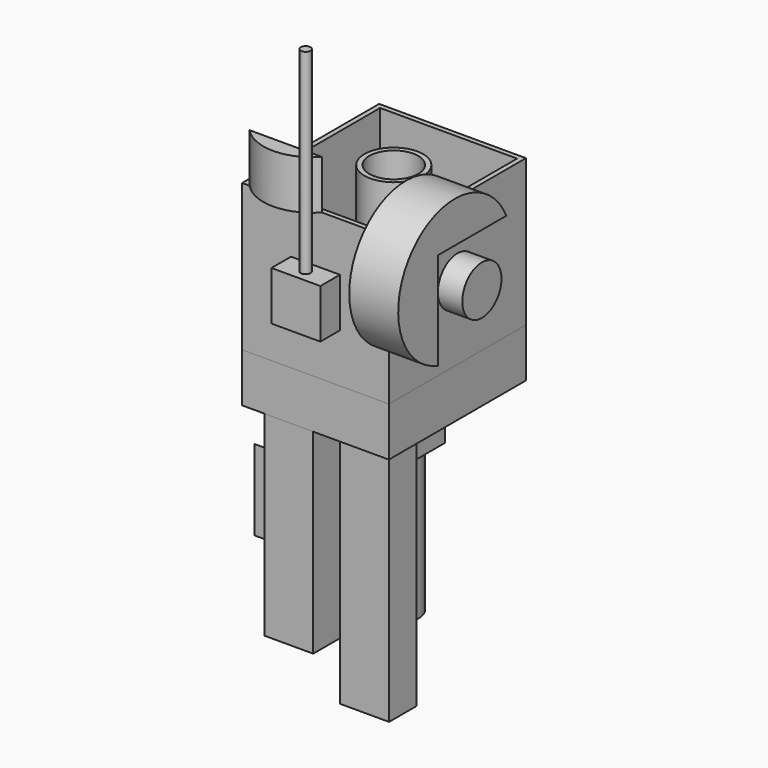
from build123d import *

# Parameters (mm, degrees)
F0_W          = 76.2
F0_H          = 76.2
F1_DEPTH      = 76.2
F3_D          = 25.4
F5_W          = 76.2
F5_H          = 76.2
F5_W_2        = 25.4
F5_H_2        = 25.4
F1_FACE1_W    = 76.2
F1_FACE1_H    = 76.2
F1_FACE2_W    = 76.2
F1_FACE2_H    = 76.2
F4_W          = 76.2
F4_H          = 76.2
F6_DEPTH      = 12.7
F7_W          = 25.4
F7_H          = 25.4
F8_DEPTH      = 12.7
F9_R          = 12.7
F10_DEPTH     = 12.7
F11_DEPTH     = 12.7
F14_DEPTH     = 25.4
F16_DEPTH     = 25.4
F17_R         = 2.54
F18_DEPTH     = 101.6
F21_W         = 25.4
F21_H         = 17.9451964796
F22_DEPTH     = 177.8
F23_W         = 25.4
F23_H         = 25.4
F24_DEPTH     = 127
F23_R         = 12.7
F25_DEPTH     = 25.4
F26_W         = 25.4
F26_H         = 25.4
F26_W_2       = 2.54
F26_H_2       = 2.54
F27_DEPTH     = 25.4
F28_T         = 2.54
F28_T3_DEPTH  = 30.48
F28_T5_DEPTH  = 30.48
F28_T7_DEPTH  = 30.48
F28_T9_DEPTH  = 30.48
F28_T11_DEPTH = 23.0251964796
F28_T13_DEPTH = 30.48
F30_DEPTH     = 25.4


# Not quite as in the source:
# - a shell that OpenCascade refuses in one call is made with other operations: the cavity is built on its own and cut out
# - the program builds the solid bodies; features that only make, move or delete a surface that nothing else refers to are left out


with BuildPart() as f1:
    # F0 (on Front) → F1 (new body)
    with BuildSketch(Plane.XZ):
        with Locations((38.1, 38.1)):
            Rectangle(F0_W, F0_H)
    extrude(amount=F1_DEPTH)

    # F3 (through all)
    with Locations(Plane.XY.offset(76.2)):
        with Locations((38.1, -38.1)):
            Hole(F3_D / 2)

    # F5 (on face) + F1_face1 (on face) + F1_face2 (on face) + F4 (on face) → F6 (join)
    with BuildSketch(Plane.XZ.offset(76.2)):
        with Locations((38.1, 38.1)):
            Rectangle(F5_W, F5_H)
        with Locations((42.7430447519, 38.5519705385)):
            Rectangle(F5_W_2, F5_H_2, mode=Mode.SUBTRACT)
        with Locations((42.7430447519, 38.5519705385)):
            Rectangle(F5_W_2, F5_H_2)
    with BuildSketch(Plane(origin=(38.1, -76.2, 38.1), x_dir=(1, 0, 0), z_dir=(0, -1, 0))):
        Rectangle(F1_FACE1_W, F1_FACE1_H)
    with BuildSketch(Plane(origin=(38.1, 0, 38.1), x_dir=(1, 0, 0), z_dir=(0, 1, 0))):
        Rectangle(F1_FACE2_W, F1_FACE2_H)
    with BuildSketch(Plane.XZ.offset(76.2)):
        with Locations((38.1, 38.1)):
            Rectangle(F4_W, F4_H)
    extrude(amount=F6_DEPTH, dir=(0, -1, 0))

    # F7 (on face) → F8 (join)
    with BuildSketch(Plane.XZ.offset(88.9)):
        with Locations((38.1, 38.1)):
            Rectangle(F7_W, F7_H)
    extrude(amount=F8_DEPTH)

    # F9 (on face) → F10 (join)
    with BuildSketch(Plane.YZ.offset(76.2)):
        with Locations((-44.45, 38.1)):
            Circle(F9_R)
    extrude(amount=F10_DEPTH)

    # F9 (on face) → F11 (join)
    with BuildSketch(Plane.YZ.offset(76.2)):
        with Locations((-44.45, 38.1)):
            Circle(F9_R)
    extrude(amount=F11_DEPTH)

    # F17 (on face) → F18 (join)
    with BuildSketch(Plane.XY.offset(50.8)):
        with Locations((38.1, -95.25)):
            Circle(F17_R)
    extrude(amount=F18_DEPTH)

    # F21 (on face) → F22 (join)
    with BuildSketch(Plane(origin=(0, 0, 25.4), x_dir=(1, 0, 0), z_dir=(0, 0, -1))):
        with Locations((54.9631331444, 69.1445562989)):
            Rectangle(F21_W, F21_H)
    extrude(amount=F22_DEPTH)

    # F23 (on face) → F24 (join)
    with BuildSketch(Plane(origin=(0, 0, 0), x_dir=(1, 0, 0), z_dir=(0, 0, -1))):
        with Locations((24.0401503026, 75.9710382342)):
            Rectangle(F23_W, F23_H)
    extrude(amount=F24_DEPTH)


with BuildPart() as f14:
    # F13 (on face) → F14 (new body)
    with BuildSketch(Plane.XY.offset(76.2)):
        with BuildLine():
            Line((41.4113799153, -88.9), (3.9465616716, -88.9))
            ThreePointArc((3.9465616716, -88.9), (22.6789707935, -97.1460835815), (41.4113799153, -88.9))
        make_face()
    extrude(amount=F14_DEPTH)


with BuildPart() as f16:
    # F15 (on face) → F16 (new body)
    with BuildSketch(Plane.YZ.offset(76.2)):
        with BuildLine():
            Line((-88.9, 76.2), (-44.45, 76.2))
            ThreePointArc((-44.45, 76.2), (-105.4397398951, 85.081047549), (-88.9, 25.7088454487))
            Line((-88.9, 25.7088454487), (-88.9, 76.2))
        make_face()
    extrude(amount=F16_DEPTH)


with BuildPart() as f24:
    # F23 (on face) → F24, piece 2 (new body)
    with BuildSketch(Plane(origin=(0, 0, 0), x_dir=(1, 0, 0), z_dir=(0, 0, -1))):
        with Locations((38.1, 38.1)):
            Circle(F23_R)
    extrude(amount=F24_DEPTH)


with BuildPart() as f25:
    # F25 (new): a face of the model
    f25_faces = [f1.part.faces().sort_by_distance(p)[0] for p in [
        (38.1, -1.1708821461, 0),
    ]]
    extrude(f25_faces, amount=F25_DEPTH)


with BuildPart() as f27:
    # F26 (on face) → F27 (new body)
    with BuildSketch(Plane(origin=(0, 0, -25.4), x_dir=(1, 0, 0), z_dir=(0, 0, -1))):
        with Locations((41.617895323, 37.7135920942)):
            Rectangle(F26_W, F26_H)
        with Locations((42.887895323, 38.9835920942)):
            Rectangle(F26_W_2, F26_H_2, mode=Mode.SUBTRACT)
    extrude(amount=F27_DEPTH)


with BuildPart() as f1_1:
    add(f1.part)

    # F28: shell of thickness 2.54, made by hand


with BuildPart() as f28_core1:
    # F28_t2: copy of F1
    add(f1_1.part)

    # the walls: a layer under each face that stays
    f28_faces = [f28_core1.faces().sort_by_distance(p)[0] for p in [
        (0, -44.45, 38.1),
        (38.1, 0, 38.1),
        (12.7, -88.9, 12.7),
        (12.7, -44.45, 0),
        (76.2, -74.0833333333, 12.7),
        (25.4, -38.1, 38.1),
        (46.5666666667, -99.4833333333, 50.8),
        (25.4, -95.25, 38.1),
        (38.1, -95.25, 25.4),
        (50.8, -95.25, 38.1),
        (11.3401503026, -75.9710382342, -63.5),
        (24.0401503026, -88.6710382342, -63.5),
        (36.7401503026, -75.9710382342, -63.5),
        (24.0401503026, -63.2710382342, -63.5),
        (67.6631331444, -69.1445562989, -76.2),
        (54.9631331444, -60.1719580591, -76.2),
        (54.9631331444, -78.1171545386, -76.2),
        (42.2631331444, -69.1445562989, -76.2),
        (82.55, -57.15, 38.1),
        (38.1, -101.6, 38.1),
        (24.0401503026, -75.9710382342, -127),
        (54.9631331444, -69.1445562989, -152.4),
        (88.9, -44.45, 38.1),
        (38.1, -95.25, 152.4),
    ]]
    thicken(f28_faces, amount=-F28_T, mode=Mode.SUBTRACT)

    # F28_s4 → F28_t3 (cut)
    with BuildSketch(Plane.YZ.offset(22.86)):
        Polygon((-88.9254, 50.8254), (-86.36, 50.8), (-86.36, 48.26), (-88.9, 48.26), align=None)
        Polygon((-88.9254, 25.3746), (-86.36, 25.4), (-86.36, 27.94), (-88.9, 27.94), align=None)
    extrude(amount=F28_T3_DEPTH, mode=Mode.SUBTRACT)

    # F28_s6 → F28_t5 (cut)
    with BuildSketch(Plane.XY.offset(22.86)):
        Polygon((25.3746, -88.9254), (25.4, -86.36), (27.94, -86.36), (27.94, -88.9), align=None)
        Polygon((50.8254, -88.9254), (50.8, -86.36), (48.26, -86.36), (48.26, -88.9), align=None)
    extrude(amount=F28_T5_DEPTH, mode=Mode.SUBTRACT)

    # F28_s8 → F28_t7 (cut)
    with BuildSketch(Plane.XZ.offset(60.7310382342)):
        Polygon((11.3147503026, -0.0254), (11.3401503026, 2.54), (13.8801503026, 2.54), (13.8801503026, 0), align=None)
        Polygon((36.7655503026, -0.0254), (36.7401503026, 2.54), (34.2001503026, 2.54), (34.2001503026, 0), align=None)
    extrude(amount=F28_T7_DEPTH, mode=Mode.SUBTRACT)

    # F28_s10 → F28_t9 (cut)
    with BuildSketch(Plane.YZ.offset(8.8001503026)):
        Polygon((-88.6964382342, -0.0254), (-88.6710382342, 2.54), (-86.1310382342, 2.54), (-86.1310382342, 0), align=None)
        Polygon((-63.2456382342, -0.0254), (-63.2710382342, 2.54), (-65.8110382342, 2.54), (-65.8110382342, 0), align=None)
    extrude(amount=F28_T9_DEPTH, mode=Mode.SUBTRACT)

    # F28_s12 → F28_t11 (cut)
    with BuildSketch(Plane.XZ.offset(57.6319580591)):
        Polygon((67.6885331444, -0.0254), (67.6631331444, 2.54), (65.1231331444, 2.54), (65.1231331444, 0), align=None)
        Polygon((42.2377331444, -0.0254), (42.2631331444, 2.54), (44.8031331444, 2.54), (44.8031331444, 0), align=None)
    extrude(amount=F28_T11_DEPTH, mode=Mode.SUBTRACT)

    # F28_s14 → F28_t13 (cut)
    with BuildSketch(Plane.YZ.offset(39.7231331444)):
        Polygon((-60.1465580591, -0.0254), (-60.1719580591, 2.54), (-62.7119580591, 2.54), (-62.7119580591, 0), align=None)
        Polygon((-78.1425545386, -0.0254), (-78.1171545386, 2.54), (-75.5771545386, 2.54), (-75.5771545386, 0), align=None)
    extrude(amount=F28_T13_DEPTH, mode=Mode.SUBTRACT)

    # F28_s15 → F28_t16 (revolve, cut)
    with BuildSketch(Plane.XY.offset(38.1)):
        Polygon((76.2254, -31.7246), (73.66, -31.75), (73.66, -34.29), (76.2, -34.29), align=None)
    revolve(axis=Axis((76.2, -44.45, 38.1), (1, 0, 0)), mode=Mode.SUBTRACT)

    # F28_s17 → F28_t18 (revolve, cut)
    with BuildSketch(Plane.XZ.offset(95.25)):
        Polygon((40.6654, 50.8254), (40.64, 48.26), (38.1, 48.26), (38.1, 50.8), align=None)
    revolve(axis=Axis((38.1, -95.25, 50.8), (0, 0, 1)), mode=Mode.SUBTRACT)


with BuildPart() as f1_2:
    add(f1_1.part)

    # what is left inside the walls is the cavity
    f28_cavity = [f28_core1.part.solids().sort_by_distance(p)[0] for p in [
        (22.8346, -38.1, 27.093333),
    ]]
    add(f28_cavity, mode=Mode.SUBTRACT)


with BuildPart() as f30:
    # F29 (on face) → F30 (new body)
    with BuildSketch(Plane(origin=(11.3401503026, 0, 0), x_dir=(0, -1, 0), z_dir=(-1, 0, 0))):
        with BuildLine():
            Line((63.2710382342, -99.802256586), (63.2710382342, -58.0201558769))
            ThreePointArc((63.2710382342, -58.0201558769), (52.3183222379, -78.9112062314), (63.2710382342, -99.802256586))
        make_face()
    extrude(amount=F30_DEPTH)


solid = Compound([f14.part, f16.part, f24.part, f25.part, f27.part, f1_2.part, f30.part])
